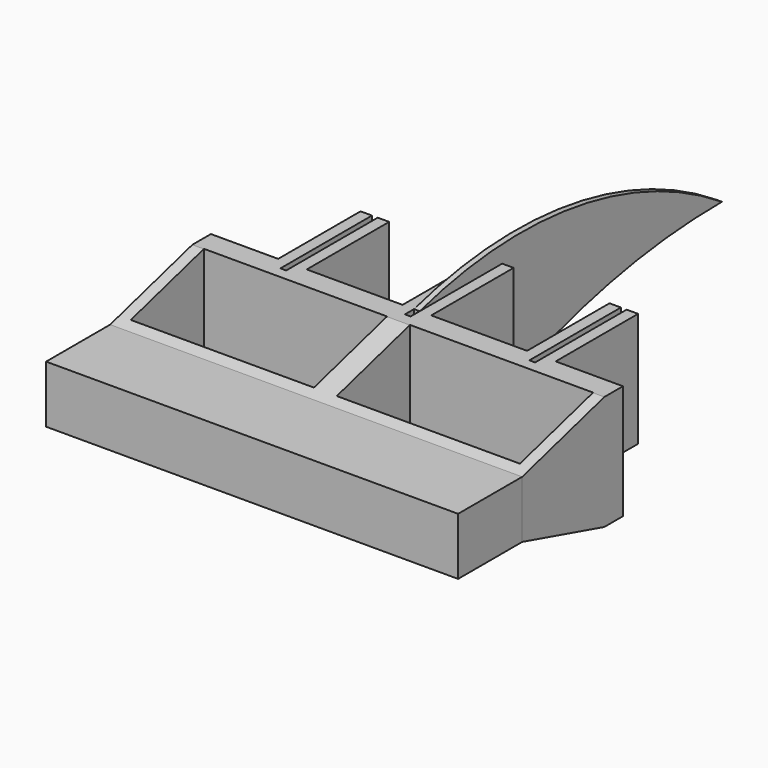
from build123d import *

# Parameters (mm, degrees)
F0_W          = 50.8
F0_H          = 25.4
F1_DEPTH      = 15.875
F1_DEPTH_BACK = 15.875
F2_DEPTH      = 7.9502
F2_DEPTH_BACK = 7.9502
F3_DEPTH      = 15.875
F3_DEPTH_BACK = 15.875
F7_DEPTH      = 57.15
F7_DEPTH_BACK = 57.15
F9_DEPTH      = 0.79375
F9_DEPTH_BACK = 0.79375


# Not quite as in the source:
# - the program builds the solid bodies; features that only make, move or delete a surface that nothing else refers to are left out


with BuildPart() as f1:
    # F0 (on Top) → F1 (new body, two sides)
    with BuildSketch(Plane.XY) as f1_sk:
        Polygon((-57.15, -3.175), (0, -3.175), (57.15, -3.175), (57.15, 28.575), (35.321875, 28.575), (33.734375, 28.575), (32.54375, 28.575), (0.79375, 28.575), (-0.79375, 28.575), (-32.54375, 28.575), (-33.734375, 28.575), (-35.321875, 28.575), (-57.15, 28.575), align=None)
        with Locations((-28.575, 12.7)):
            Rectangle(F0_W, F0_H, mode=Mode.SUBTRACT)
        with Locations((28.575, 12.7)):
            Rectangle(F0_W, F0_H, mode=Mode.SUBTRACT)
        Polygon((-57.15, 31.75), (-57.15, 28.575), (-35.321875, 28.575), (-35.321875, 60.325), (-38.496875, 60.325), (-38.496875, 31.75), align=None)
        Polygon((35.321875, 28.575), (57.15, 28.575), (57.15, 31.75), (38.496875, 31.75), (38.496875, 60.325), (35.321875, 60.325), align=None)
        Polygon((32.54375, 28.575), (33.734375, 28.575), (33.734375, 60.325), (30.559375, 60.325), (30.559375, 31.75), (17.2640625, 31.75), (3.96875, 31.75), (3.96875, 60.325), (0.79375, 60.325), (0.79375, 28.575), align=None)
        Polygon((-33.734375, 60.325), (-33.734375, 28.575), (-32.54375, 28.575), (-0.79375, 28.575), (-0.79375, 60.325), (-3.96875, 60.325), (-3.96875, 31.75), (-17.2640625, 31.75), (-30.559375, 31.75), (-30.559375, 60.325), align=None)
    extrude(amount=F1_DEPTH)
    extrude(f1_sk.sketch, amount=-F1_DEPTH_BACK)

    # F0 (on Top) → F3 (join, two sides)
    with BuildSketch(Plane.XY) as f3_sk:
        Polygon((-33.734375, 60.325), (-33.734375, 28.575), (-32.54375, 28.575), (-0.79375, 28.575), (-0.79375, 60.325), (-3.96875, 60.325), (-3.96875, 31.75), (-17.2640625, 31.75), (-30.559375, 31.75), (-30.559375, 60.325), align=None)
        Polygon((32.54375, 28.575), (33.734375, 28.575), (33.734375, 60.325), (30.559375, 60.325), (30.559375, 31.75), (17.2640625, 31.75), (3.96875, 31.75), (3.96875, 60.325), (0.79375, 60.325), (0.79375, 28.575), align=None)
    extrude(amount=F3_DEPTH)
    extrude(f3_sk.sketch, amount=-F3_DEPTH_BACK)

    # F6 (on Right) → F7 (cut, two sides)
    with BuildSketch(Plane.YZ) as f7_sk:
        Polygon((25.4, -15.9004), (-3.175, -7.9502), (-3.175, -15.9004), align=None)
        Polygon((-3.175, 15.9004), (-3.175, 7.9502), (25.4, 15.9004), align=None)
    extrude(amount=-F7_DEPTH, mode=Mode.SUBTRACT)
    extrude(f7_sk.sketch, amount=F7_DEPTH_BACK, mode=Mode.SUBTRACT)


with BuildPart() as f2:
    # F0 (on Top) → F2 (new body, two sides)
    with BuildSketch(Plane.XY) as f2_sk:
        Polygon((57.15, -3.175), (0, -3.175), (-57.15, -3.175), (-57.15, -25.4), (57.15, -25.4), align=None)
    extrude(amount=F2_DEPTH)
    extrude(f2_sk.sketch, amount=-F2_DEPTH_BACK)


with BuildPart() as f9:
    # F8 (on Right) → F9 (new body, two sides)
    with BuildSketch(Plane.YZ) as f9_sk:
        with BuildLine():
            ThreePointArc((60.325, -15.875), (97.606959116, -4.0109037567), (136.525, 0))
            ThreePointArc((136.525, 0), (85.8723958548, 19.3878126418), (31.75, 15.875))
            Line((31.75, 15.875), (31.75, -15.875))
            Line((31.75, -15.875), (60.325, -15.875))
        make_face()
    extrude(amount=F9_DEPTH)
    extrude(f9_sk.sketch, amount=-F9_DEPTH_BACK)


solid = Compound([f1.part, f2.part, f9.part])
